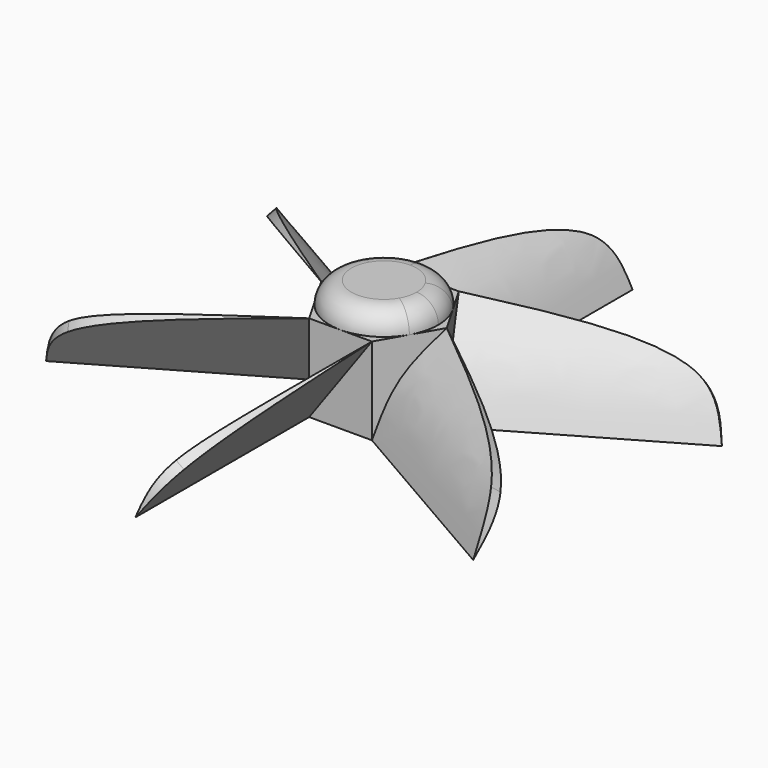
from build123d import *

# Parameters (mm, degrees)
F1_DEPTH  = 20
F3_DEPTH  = 50
F5_DEPTH  = 50
F7_DEPTH  = 50
F9_DEPTH  = 50
F11_DEPTH = 50
F13_DEPTH = 50
F15_DEPTH = 25
F17_DEPTH = 25
F19_DEPTH = 25
F21_DEPTH = 25
F23_DEPTH = 25
F25_DEPTH = 25
F27_DEPTH = 5
F28_R     = 4.99999
F29_R     = 1.5
F30_DEPTH = 16.1


# Not quite as in the source:
# - a fillet or chamfer is up to 0.001 mm smaller than in the source, because OpenCascade refuses the exact size


with BuildPart() as f1:
    # F0 (on Top) → F1 (new body)
    with BuildSketch(Plane.XY):
        Polygon((-7.2168783649, 12.5), (-14.4337567297, 0), (-7.2168783649, -12.5), (7.2168783649, -12.5), (14.4337567297, 0), (7.2168783649, 12.5), align=None)
    extrude(amount=F1_DEPTH)

    # F2 (on face) → F3 (join)
    with BuildSketch(Plane.XZ.offset(12.5)):
        with BuildLine():
            Line((0, 10), (7.2168783649, 20))
            add(Edge.make_bspline(
                [(7.2168783649, 20), (3.8943965132, 17.3283502948), (0.5892440485, 14.6441941819), (-1.8163820731, 11.3108608486)],
                knots=[0, 0, 0, 0, 0.5, 0.5, 0.5, 0.5], degree=3))
            Line((-1.8163820731, 11.3108608486), (0, 10))
        make_face()
        with BuildLine():
            Line((-7.2168783649, 0), (0, 10))
            Line((0, 10), (-1.8163820731, 11.3108608486))
            add(Edge.make_bspline(
                [(-1.8163820731, 11.3108608486), (-4.2220081948, 7.9775275153), (-5.7281079733, 3.9950169615), (-7.2168783649, 0)],
                knots=[0.5, 0.5, 0.5, 0.5, 1, 1, 1, 1], degree=3))
        make_face()
    extrude(amount=F3_DEPTH)

    # F4 (on face) → F5 (join)
    with BuildSketch(Plane(origin=(10.8253175473, -6.25, 0), x_dir=(0.5, 0.8660254038, 0), z_dir=(0.8660254038, -0.5, 0))):
        with BuildLine():
            Line((-7.2168783649, 0), (7.2168783649, 20))
            add(Edge.make_bspline(
                [(7.2168783649, 20), (3.8943965132, 17.3283502948), (-2.7159084163, 11.960038069), (-5.7281079733, 3.9950169615), (-7.2168783649, 0)],
                knots=[0, 0, 0, 0, 0.5, 1, 1, 1, 1], degree=3))
        make_face()
    extrude(amount=F5_DEPTH)

    # F6 (on face) → F7 (join)
    with BuildSketch(Plane(origin=(10.8253175473, 6.25, 0), x_dir=(-0.5, 0.8660254038, 0), z_dir=(0.8660254038, 0.5, 0))):
        with BuildLine():
            Line((-7.2168783649, 0), (7.2168783649, 20))
            add(Edge.make_bspline(
                [(7.2168783649, 20), (3.8943965132, 17.3283502948), (-2.7159084163, 11.960038069), (-5.7281079733, 3.9950169615), (-7.2168783649, 0)],
                knots=[0, 0, 0, 0, 0.5, 1, 1, 1, 1], degree=3))
        make_face()
    extrude(amount=F7_DEPTH)

    # F8 (on face) → F9 (join)
    with BuildSketch(Plane(origin=(0, 12.5, 0), x_dir=(-1, 0, 0), z_dir=(0, 1, 0))):
        with BuildLine():
            Line((-7.183146663, 0), (7.2506100667, 20))
            add(Edge.make_bspline(
                [(7.2506100667, 20), (3.9281282151, 17.3283502948), (-2.6821767144, 11.960038069), (-5.6943762714, 3.9950169615), (-7.183146663, 0)],
                knots=[0, 0, 0, 0, 0.5, 1, 1, 1, 1], degree=3))
        make_face()
    extrude(amount=F9_DEPTH)

    # F10 (on face) → F11 (join)
    with BuildSketch(Plane(origin=(-10.8253175473, 6.25, 0), x_dir=(-0.5, -0.8660254038, 0), z_dir=(-0.8660254038, 0.5, 0))):
        with BuildLine():
            Line((-7.2168783649, 0), (7.2168783649, 20))
            add(Edge.make_bspline(
                [(7.2168783649, 20), (3.8943965132, 17.3283502948), (-2.7159084163, 11.960038069), (-5.7281079733, 3.9950169615), (-7.2168783649, 0)],
                knots=[0, 0, 0, 0, 0.5, 1, 1, 1, 1], degree=3))
        make_face()
    extrude(amount=F11_DEPTH)

    # F12 (on face) → F13 (join)
    with BuildSketch(Plane(origin=(-10.8253175473, -6.25, 0), x_dir=(0.5, -0.8660254038, 0), z_dir=(-0.8660254038, -0.5, 0))):
        with BuildLine():
            Line((-7.2168782353, 0), (7.2168784944, 20))
            add(Edge.make_bspline(
                [(7.2168784944, 20), (3.8943966428, 17.3283502948), (-2.7159082867, 11.960038069), (-5.7281078437, 3.9950169615), (-7.2168782353, 0)],
                knots=[0, 0, 0, 0, 0.5, 1, 1, 1, 1], degree=3))
        make_face()
    extrude(amount=F13_DEPTH)

    # F14 (on face) → F15 (cut)
    with BuildSketch(Plane(origin=(-2.3726722966, 4.1095889673, 3.4246574728), x_dir=(0.914120582, 0.3114695001, 0.2595579168), z_dir=(0.405442427, -0.7022468832, -0.585205736))):
        with BuildLine():
            Line((-52.6686272502, 39.3713406512), (-56.6160705917, 27.6879752855))
            Line((-56.6160705917, 27.6879752855), (-51.879138611, 26.0875142863))
            add(Edge.make_bspline(
                [(-51.879138611, 26.0875142863), (-42.9404048496, 29.8743142581), (-24.1198561583, 26.6205224229), (-5.299307467, 23.3667305878)],
                knots=[0.3481274936, 0.3481274936, 0.3481274936, 0.3481274936, 1, 1, 1, 1], degree=3))
            Line((-5.2993074428, 23.3667306596), (-52.6686272502, 39.3713406512))
        make_face()
        with BuildLine():
            Line((-51.879138611, 26.0875142863), (-56.6160705917, 27.6879752855))
            Line((-56.6160705917, 27.6879752855), (-60.5635138847, 16.0046100634))
            add(Edge.make_bspline(
                [(-60.563513909, 16.0046099916), (-58.608157235, 20.034906453), (-56.6528005609, 24.0652029143), (-51.879138611, 26.0875142863)],
                knots=[0, 0, 0, 0, 0.3481274936, 0.3481274936, 0.3481274936, 0.3481274936], degree=3))
        make_face()
    extrude(amount=-F15_DEPTH, mode=Mode.SUBTRACT)

    # F16 (on face) → F17 (cut)
    with BuildSketch(Plane(origin=(-4.7453446783, 0, 3.4246575342), x_dir=(0, 1, 0), z_dir=(0.8108848541, 0, -0.585205736))):
        with BuildLine():
            Line((-62.5, 20.4410556966), (-62.5, 8.1088485408))
            Line((-62.5, 8.1088485408), (-57.5, 8.1088485408))
            add(Edge.make_bspline(
                [(-57.5, 8.1088485408), (-50.2436903689, 14.5576302724), (-31.3718451845, 17.4993429845), (-12.5, 20.4410556966)],
                knots=[0.3481274936, 0.3481274936, 0.3481274936, 0.3481274936, 1, 1, 1, 1], degree=3))
            Line((-12.5, 20.4410556966), (-62.5, 20.4410556966))
        make_face()
        with BuildLine():
            Line((-57.5, 8.1088485408), (-62.5, 8.1088485408))
            Line((-62.5, 8.1088485408), (-62.5, -4.223358615))
            add(Edge.make_bspline(
                [(-62.5, -4.223358615), (-61.9375881477, 0.2207838442), (-61.3751762953, 4.6649263034), (-57.5, 8.1088485408)],
                knots=[0, 0, 0, 0, 0.3481274936, 0.3481274936, 0.3481274936, 0.3481274936], degree=3))
        make_face()
    extrude(amount=-F17_DEPTH, mode=Mode.SUBTRACT)

    # F18 (on face) → F19 (cut)
    with BuildSketch(Plane(origin=(-2.3726723391, -4.1095890411, 3.4246575342), x_dir=(-0.914120582, 0.3114695001, -0.2595579168), z_dir=(0.405442427, 0.7022468832, -0.585205736))):
        with BuildLine():
            Line((-65.7546722441, -0.6401843997), (-61.8072289268, -12.3235496935))
            Line((-61.8072289268, -12.3235496935), (-57.070296946, -10.7230886944))
            add(Edge.make_bspline(
                [(-57.070296946, -10.7230886944), (-52.259972646, -2.2909124977), (-35.3226625414, 6.5367565471), (-18.3853524367, 15.3644255919)],
                knots=[0.3481274936, 0.3481274936, 0.3481274936, 0.3481274936, 1, 1, 1, 1], degree=3))
            Line((-18.3853524367, 15.3644255919), (-65.7546722441, -0.6401843997))
        make_face()
        with BuildLine():
            Line((-57.070296946, -10.7230886944), (-61.8072289268, -12.3235496935))
            Line((-61.8072289268, -12.3235496935), (-57.8597856095, -24.0069149874))
            add(Edge.make_bspline(
                [(-57.8597856095, -24.0069149874), (-58.7494996077, -19.616571232), (-59.6392136059, -15.2262274766), (-57.070296946, -10.7230886944)],
                knots=[0, 0, 0, 0, 0.3481274936, 0.3481274936, 0.3481274936, 0.3481274936], degree=3))
        make_face()
    extrude(amount=-F19_DEPTH, mode=Mode.SUBTRACT)

    # F20 (on face) → F21 (cut)
    with BuildSketch(Plane(origin=(2.3726723391, -4.1095890411, 3.4246575342), x_dir=(-0.914120582, -0.3114695001, 0.2595579168), z_dir=(-0.405442427, 0.7022468832, -0.585205736))):
        with BuildLine():
            Line((-52.6686272744, 39.3713405794), (-56.6160705917, 27.6879752855))
            Line((-56.6160705917, 27.6879752855), (-51.879138611, 26.0875142863))
            add(Edge.make_bspline(
                [(-51.879138611, 26.0875142863), (-42.9404048496, 29.8743142581), (-24.1198561583, 26.6205224229), (-5.299307467, 23.3667305878)],
                knots=[0.3481274936, 0.3481274936, 0.3481274936, 0.3481274936, 1, 1, 1, 1], degree=3))
            Line((-5.299307467, 23.3667305878), (-52.6686272744, 39.3713405794))
        make_face()
        with BuildLine():
            Line((-51.879138611, 26.0875142863), (-56.6160705917, 27.6879752855))
            Line((-56.6160705917, 27.6879752855), (-60.563513909, 16.0046099916))
            add(Edge.make_bspline(
                [(-60.563513909, 16.0046099916), (-58.608157235, 20.034906453), (-56.6528005609, 24.0652029143), (-51.879138611, 26.0875142863)],
                knots=[0, 0, 0, 0, 0.3481274936, 0.3481274936, 0.3481274936, 0.3481274936], degree=3))
        make_face()
    extrude(amount=-F21_DEPTH, mode=Mode.SUBTRACT)

    # F22 (on face) → F23 (cut)
    with BuildSketch(Plane(origin=(4.7231649291, 0, 3.4086506791), x_dir=(0, -1, 0), z_dir=(-0.8108848541, 0, -0.585205736))):
        with BuildLine():
            Line((-62.5, 20.460795682), (-62.5, 8.1285885262))
            Line((-62.5, 8.1285885262), (-57.5, 8.1285885262))
            add(Edge.make_bspline(
                [(-57.5, 8.1285885262), (-50.2436903689, 14.5773702578), (-31.3718451845, 17.5190829699), (-12.5, 20.460795682)],
                knots=[0.3481274936, 0.3481274936, 0.3481274936, 0.3481274936, 1, 1, 1, 1], degree=3))
            Line((-12.5, 20.460795682), (-62.5, 20.460795682))
        make_face()
        with BuildLine():
            Line((-57.5, 8.1285885262), (-62.5, 8.1285885262))
            Line((-62.5, 8.1285885262), (-62.5, -4.2036186296))
            add(Edge.make_bspline(
                [(-62.5, -4.2036186296), (-61.9375881477, 0.2405238296), (-61.3751762953, 4.6846662888), (-57.5, 8.1285885262)],
                knots=[0, 0, 0, 0, 0.3481274936, 0.3481274936, 0.3481274936, 0.3481274936], degree=3))
        make_face()
    extrude(amount=-F23_DEPTH, mode=Mode.SUBTRACT)

    # F24 (on face) → F25 (cut)
    with BuildSketch(Plane(origin=(2.3726723391, 4.1095890411, 3.4246575342), x_dir=(0.914120582, -0.3114695001, -0.2595579168), z_dir=(-0.405442427, -0.7022468832, -0.585205736))):
        with BuildLine():
            Line((-65.7546722441, -0.6401843997), (-61.8072289268, -12.3235496935))
            Line((-61.8072289268, -12.3235496935), (-57.070296946, -10.7230886944))
            add(Edge.make_bspline(
                [(-57.070296946, -10.7230886944), (-52.259972646, -2.2909124977), (-35.3226625414, 6.5367565471), (-18.3853524367, 15.3644255919)],
                knots=[0.3481274936, 0.3481274936, 0.3481274936, 0.3481274936, 1, 1, 1, 1], degree=3))
            Line((-18.3853524367, 15.3644255919), (-65.7546722441, -0.6401843997))
        make_face()
        with BuildLine():
            Line((-57.070296946, -10.7230886944), (-61.8072289268, -12.3235496935))
            Line((-61.8072289268, -12.3235496935), (-57.8597856095, -24.0069149874))
            add(Edge.make_bspline(
                [(-57.8597856095, -24.0069149874), (-58.7494996077, -19.616571232), (-59.6392136059, -15.2262274766), (-57.070296946, -10.7230886944)],
                knots=[0, 0, 0, 0, 0.3481274936, 0.3481274936, 0.3481274936, 0.3481274936], degree=3))
        make_face()
    extrude(amount=-F25_DEPTH, mode=Mode.SUBTRACT)

    # F26 (on face) → F27 (join)
    with BuildSketch(Plane.XY.offset(20)):
        with BuildLine():
            ThreePointArc((10.8253174264, -6.2500002094), (12.0740727973, -3.2352381805), (12.5, 0))
            ThreePointArc((12.5, 0), (12.0740728368, 3.2352380332), (10.825317579, 6.2499999451))
            ThreePointArc((10.825317579, 6.2499999451), (6.2500000275, 10.8253175315), (0, 12.5))
            ThreePointArc((0, 12.5), (-6.2500001608, 10.8253174545), (-10.825317733, 6.2499996783))
            ThreePointArc((-10.825317733, 6.2499996783), (-12.5, -1.905e-07), (-10.8253175425, -6.2500000083))
            ThreePointArc((-10.8253175425, -6.2500000083), (-6.2499999958, -10.8253175497), (0, -12.5))
            ThreePointArc((0, -12.5), (6.2499998953, -10.8253176077), (10.8253174264, -6.2500002094))
        make_face()
    extrude(amount=F27_DEPTH)

    # F28 (radius 5 in the source; OpenCascade refuses exactly that, so slightly less here)
    f28_edges = [f1.edges().sort_by_distance(p)[0] for p in [
        (10.825318, 6.25, 25),
    ]]
    fillet(f28_edges, radius=F28_R)

    # F29 (on face) → F30 (cut)
    with BuildSketch(Plane(origin=(0, 0, 0), x_dir=(1, 0, 0), z_dir=(0, 0, -1))):
        Circle(F29_R)
    extrude(amount=-F30_DEPTH, mode=Mode.SUBTRACT)


solid = f1.part
